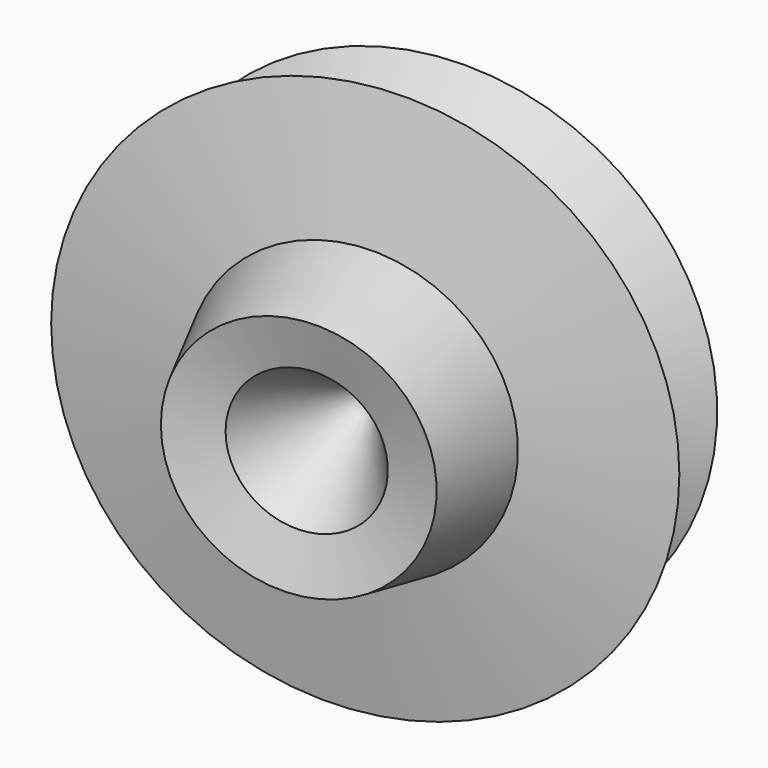
from build123d import *


with BuildPart() as f1:
    # F0 (on Top) → F1 (revolve)
    with BuildSketch(Plane.XY):
        Polygon((-23.3715903014, 33.6437821388), (-24.313993752, 26.2930374593), (-49.3819080293, 13.6648416519), (-29.7799296677, -4.0523321368), (-60.1252987981, -5.37169585), (-35.6228277087, -16.3035690784), (-60.5022609234, -31.7589752376), (-28.8375262171, -31.0050528497), (-18.8480559736, -50.9839951992), (-7.7277040109, -45.5180555582), (3.5811301786, -14.4187640399), (-11.3088339567, 61.16194278), (-20.7328628749, 47.5913472474), (-17.5286922604, 33.4553010762), align=None)
    revolve(axis=Axis((-3.863851889, 23.3715893701, 0), (-0.1932921582, 0.9811412445, 0)))


solid = f1.part
